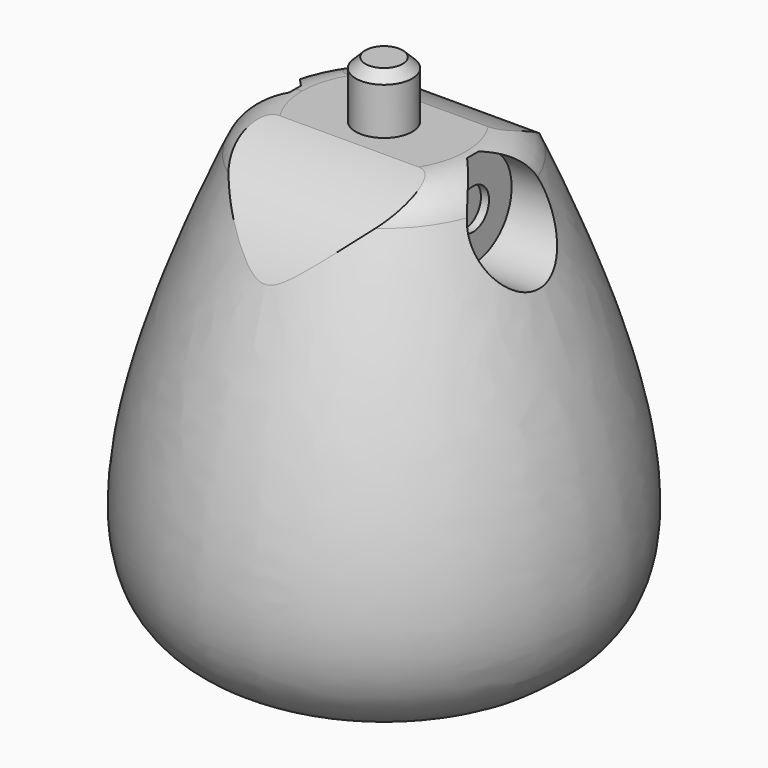
from build123d import *

# Parameters (mm, degrees)
F3_R          = 4
F4_DEPTH      = 3
F5_R          = 1.25
F6_DEPTH      = 2
F7_R          = 1.25
F8_DEPTH      = 2
F10_DEPTH     = 12.5
F11_T4_ANGLE  = 62.5690664244
F11_S5_R      = 10.55
F11_T6_DEPTH  = 7
F11_T10_ANGLE = 125.1442226545
F11_S11_R     = 10.55
F11_T12_DEPTH = 10
F11_T16_ANGLE = 62.5690664244
F11_S17_R     = 10.55
F11_T18_DEPTH = 7
F12_R         = 1.75
F13_DEPTH     = 3.5
F14_SIZE      = 0.6
F15_R         = 1.25
F16_DEPTH     = 3.3534363587
F19_R         = 1.25
F20_DEPTH     = 5
F21_R         = 3
F22_DEPTH     = 4.5
F23_R         = 1.25
F24_DEPTH     = 8
F25_R         = 3
F26_DEPTH     = 4.5


# Not quite as in the source:
# - a fillet or chamfer that OpenCascade refuses, or shapes differently, is made with other operations: its cross-section is extruded or revolved along the edge and cut away or added


with BuildPart() as f2:
    # F1 (on Front) → F2 (revolve)
    with BuildSketch(Plane.XZ):
        with BuildLine():
            Line((0, 29), (-7, 29))
            add(Edge.make_bspline(
                [(0, 0), (-5.317841365, 0), (-8.4305850004, 0.3570766518), (-14.8822587004, 4.4570633142), (-13.316672088, 15.36842657), (-7, 29)],
                knots=[0, 0, 0, 0, 0.2945682266, 0.5047389267, 1, 1, 1, 1], degree=3))
            Line((0, 0), (0, 29))
        make_face()
    revolve(axis=Axis((0, 0, 7.1166679263), (0, 0, -1)))

    # F3 (on Top) → F4 (cut)
    with BuildSketch(Plane.XY):
        with Locations((-7.6, 0)):
            Circle(F3_R)
        with Locations((7.6, 0)):
            Circle(F3_R)
    extrude(amount=F4_DEPTH, mode=Mode.SUBTRACT)

    # F5 (on face) → F6 (cut)
    with BuildSketch(Plane(origin=(0, 0, 3), x_dir=(1, 0, 0), z_dir=(0, 0, -1))):
        with Locations((7.6, 0)):
            Circle(F5_R)
    extrude(amount=-F6_DEPTH, mode=Mode.SUBTRACT)

    # F7 (on face) → F8 (cut)
    with BuildSketch(Plane(origin=(0, 0, 3), x_dir=(1, 0, 0), z_dir=(0, 0, -1))):
        with Locations((-7.6, 0)):
            Circle(F7_R)
    extrude(amount=-F8_DEPTH, mode=Mode.SUBTRACT)

    # F9 (on Right) → F10 (cut, symmetric)
    with BuildSketch(Plane.YZ):
        with BuildLine():
            Line((-10.1144698329, 31.8), (-10.1144698329, 21.8))
            ThreePointArc((-10.1144698329, 21.8), (0, 29.35), (10.1144698329, 21.8))
            Line((10.1144698329, 21.8), (10.1144698329, 31.8))
            Line((10.1144698329, 31.8), (-10.1144698329, 31.8))
        make_face()
    extrude(amount=F10_DEPTH, both=True, mode=Mode.SUBTRACT)

    # F11: fillet of radius 3 on 3 edges, made by hand


with BuildPart() as f11_tool2:
    # F11_s3 → F11_t4 (revolve)
    with BuildSketch(Plane.XZ):
        with BuildLine():
            ThreePointArc((-5.0697196206, 29), (-6.7017587776, 28.5172302616), (-7.8085318567, 27.2242987933))
            Line((-7.8085318567, 27.2242987933), (-7.8633081014, 27.2487847692))
            ThreePointArc((-7.8633081014, 27.2487847692), (-7.4618780859, 28.1383864481), (-7.0544392435, 29.0252263506))
            Line((-7.0544392435, 29.0252263506), (-7, 29.06))
            Line((-7, 29.06), (-5.0697196206, 29.06))
            Line((-5.0697196206, 29.06), (-5.0697196206, 29))
        make_face()
    revolve(axis=Axis((0, 0, 29), (0, 0, -1)), revolution_arc=F11_T4_ANGLE)

    # F11_s5 → F11_t6 (intersect, symmetric)
    with BuildSketch(Plane.YZ.offset(-5.5)):
        with Locations((0, 18.8)):
            Circle(F11_S5_R)
    extrude(amount=F11_T6_DEPTH, both=True, mode=Mode.INTERSECT)


with BuildPart() as f2_1:
    add(f2.part)

    # F11_t1: cut F11_tool2
    add(f11_tool2.part, mode=Mode.SUBTRACT)


with BuildPart() as f11_tool8:
    # F11_s9 → F11_t10 (revolve)
    with BuildSketch(Plane(origin=(0, 0, 0), x_dir=(0, 0, 1), z_dir=(-0.8875912781, 0.4606318736, 0))):
        with BuildLine():
            ThreePointArc((29, 5.0697196206), (28.5172302616, 6.7017587776), (27.2242987933, 7.8085318567))
            Line((27.2242987933, 7.8085318567), (27.2487847692, 7.8633081014))
            ThreePointArc((27.2487847692, 7.8633081014), (28.1383864481, 7.4618780859), (29.0252263506, 7.0544392435))
            Line((29.0252263506, 7.0544392435), (29.06, 7))
            Line((29.06, 7), (29.06, 5.0697196206))
            Line((29.06, 5.0697196206), (29, 5.0697196206))
        make_face()
    revolve(axis=Axis((0, 0, 29), (0, 0, -1)), revolution_arc=F11_T10_ANGLE)

    # F11_s11 → F11_t12 (intersect, symmetric)
    with BuildSketch(Plane.YZ.offset(5.3)):
        with Locations((0, 18.8)):
            Circle(F11_S11_R)
    extrude(amount=F11_T12_DEPTH, both=True, mode=Mode.INTERSECT)


with BuildPart() as f2_2:
    add(f2_1.part)

    # F11_t7: cut F11_tool8
    add(f11_tool8.part, mode=Mode.SUBTRACT)


with BuildPart() as f11_tool14:
    # F11_s15 → F11_t16 (revolve)
    with BuildSketch(Plane(origin=(0, 0, 0), x_dir=(0, 0, 1), z_dir=(0.8875667972, -0.4606790428, 0))):
        with BuildLine():
            ThreePointArc((29, 5.0697196206), (28.5172302616, 6.7017587776), (27.2242987933, 7.8085318567))
            Line((27.2242987933, 7.8085318567), (27.2487847692, 7.8633081014))
            ThreePointArc((27.2487847692, 7.8633081014), (28.1383864481, 7.4618780859), (29.0252263506, 7.0544392435))
            Line((29.0252263506, 7.0544392435), (29.06, 7))
            Line((29.06, 7), (29.06, 5.0697196206))
            Line((29.06, 5.0697196206), (29, 5.0697196206))
        make_face()
    revolve(axis=Axis((0, 0, 29), (0, 0, -1)), revolution_arc=F11_T16_ANGLE)

    # F11_s17 → F11_t18 (intersect, symmetric)
    with BuildSketch(Plane.YZ.offset(-5.5)):
        with Locations((0, 18.8)):
            Circle(F11_S17_R)
    extrude(amount=F11_T18_DEPTH, both=True, mode=Mode.INTERSECT)


with BuildPart() as f2_3:
    add(f2_2.part)

    # F11_t13: cut F11_tool14
    add(f11_tool14.part, mode=Mode.SUBTRACT)

    # F12 (on face) → F13 (join)
    with BuildSketch(Plane.XY.offset(29)):
        Circle(F12_R)
    extrude(amount=F13_DEPTH)

    # F14
    f14_edges = [f2_3.edges().sort_by_distance(p)[0] for p in [
        (-1.75, 0, 32.5),
    ]]
    chamfer(f14_edges, length=F14_SIZE)

    # F15 (on offset) → F16 (cut, through all)
    with BuildSketch(Plane.XZ.offset(-10)):
        with Locations((0, 7)):
            Circle(F15_R)
    extrude(amount=-F16_DEPTH, mode=Mode.SUBTRACT)

    # F19 (on offset) → F20 (cut)
    with BuildSketch(Plane.YZ.offset(10)):
        with Locations((0, 26)):
            Circle(F19_R)
    extrude(amount=-F20_DEPTH, mode=Mode.SUBTRACT)

    # F21 (on offset) → F22 (cut)
    with BuildSketch(Plane.YZ.offset(10)):
        with Locations((0, 26)):
            Circle(F21_R)
    extrude(amount=-F22_DEPTH, mode=Mode.SUBTRACT)

    # F23 (on offset) → F24 (cut)
    with BuildSketch(Plane.YZ.offset(-10)):
        with Locations((0, 26)):
            Circle(F23_R)
    extrude(amount=F24_DEPTH, mode=Mode.SUBTRACT)

    # F25 (on offset) → F26 (cut)
    with BuildSketch(Plane.YZ.offset(-10)):
        with Locations((0, 26)):
            Circle(F25_R)
    extrude(amount=F26_DEPTH, mode=Mode.SUBTRACT)


solid = f2_3.part
